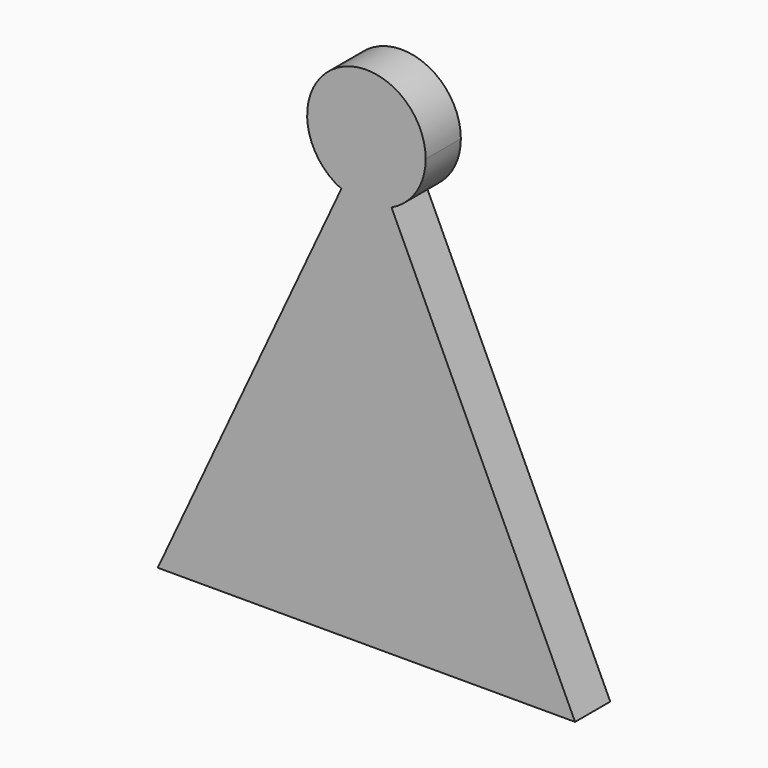
from build123d import *

# Parameters (mm, degrees)
F1_DEPTH = 4.7


with BuildPart() as f1:
    # F0 (on Front) → F1 (new body)
    with BuildSketch(Plane.XZ):
        with BuildLine():
            Line((-47.77017605, 45.9924270552), (-67.3986524343, 3.9423387498))
            Line((-67.3986524343, 3.9423387498), (-22.7815322578, 3.9423387498))
            Line((-22.7815322578, 3.9423387498), (-42.4100088013, 45.9924270633))
            ThreePointArc((-42.4100088013, 45.9924270633), (-45.0900924247, 45.3977122077), (-47.77017605, 45.9924270552))
        make_face()
        with BuildLine():
            ThreePointArc((-38.753834, 51.7339706421), (-48.4935075231, 57.0785881851), (-47.77017605, 45.9924270552))
            Line((-47.77017605, 45.9924270552), (-45.0900924343, 51.7339706421))
            Line((-45.0900924343, 51.7339706421), (-42.4100088013, 45.9924270633))
            ThreePointArc((-42.4100088013, 45.9924270633), (-39.7454748862, 48.3305555615), (-38.753834, 51.7339706421))
        make_face()
        with BuildLine():
            Line((-45.0900924343, 51.7339706421), (-47.77017605, 45.9924270552))
            ThreePointArc((-47.77017605, 45.9924270552), (-45.0900924247, 45.3977122077), (-42.4100088013, 45.9924270633))
            Line((-42.4100088013, 45.9924270633), (-45.0900924343, 51.7339706421))
        make_face()
    extrude(amount=F1_DEPTH)


solid = f1.part
